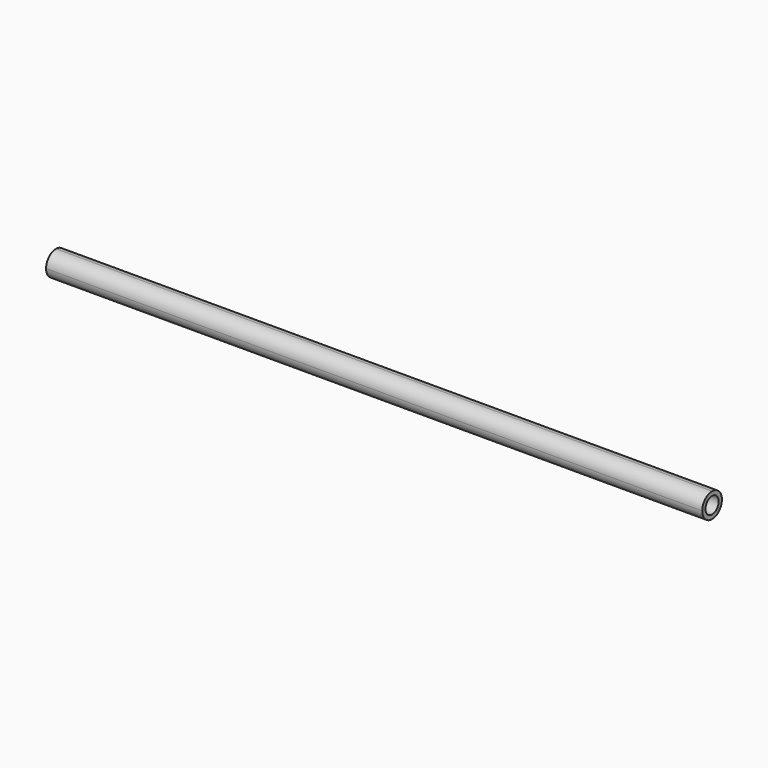
from build123d import *

# Parameters (mm, degrees)
F0_W     = 160
F0_H     = 6
F1_DEPTH = 6
F2_R     = 2.99999
F4_D     = 4


# Not quite as in the source:
# - a fillet or chamfer is up to 0.001 mm smaller than in the source, because OpenCascade refuses the exact size


with BuildPart() as f1:
    # F0 (on Top) → F1 (new body)
    with BuildSketch(Plane.XY):
        with Locations((0.9389727563, 14.3314650139)):
            Rectangle(F0_W, F0_H)
    extrude(amount=F1_DEPTH)

    # F2 (radius 3 in the source; OpenCascade refuses exactly that, so slightly less here)
    f2_edges = [f1.edges().sort_by_distance(p)[0] for p in [
        (0.938973, 17.331465, 6),
        (0.938973, 11.331465, 6),
        (0.938973, 17.331465, 0),
        (0.938973, 11.331465, 0),
    ]]
    fillet(f2_edges, radius=F2_R)

    # F4 (through all)
    with Locations(Plane.YZ.offset(80.9389727563)):
        with Locations((14.3314650139, 3)):
            Hole(F4_D / 2)


solid = f1.part
